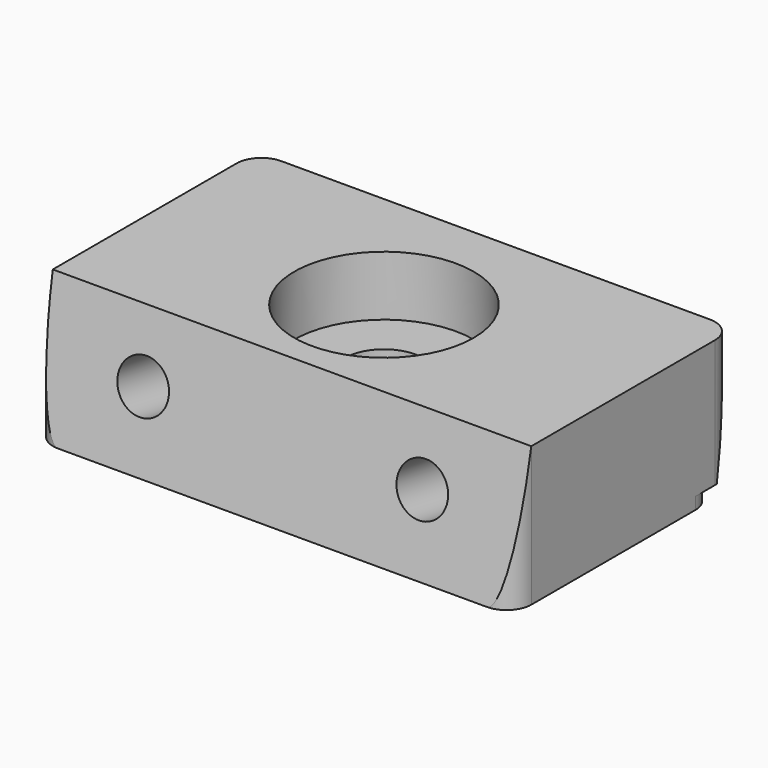
from build123d import *

# Parameters (mm, degrees)
F0_W           = 60.96
F0_H           = 35.56
F1_DEPTH       = 17.78
F2_R           = 3.175
F4_DEPTH       = 60.961
F6_D           = 10.0838
F6_DEPTH       = 23.2918
F6_CBORE_D     = 22.86
F6_CBORE_DEPTH = 7.62
F6_TIP         = 3.0294791551
F7_T1_DEPTH    = 9.4615000248
F9_D           = 6.5278
F9_DEPTH       = 23.2833333333
F9_TIP         = 1.9611489744


# Not quite as in the source:
# - a fillet or chamfer that OpenCascade refuses, or shapes differently, is made with other operations: its cross-section is extruded or revolved along the edge and cut away or added
# - a feature names something its author has since deleted; it is built from what else it names


with BuildPart() as f1:
    # F0 (on Top) → F1 (new body)
    with BuildSketch(Plane.XY):
        with Locations((30.48, 17.78)):
            Rectangle(F0_W, F0_H)
    extrude(amount=F1_DEPTH)

    # F2
    f2_edges = [f1.edges().sort_by_distance(p)[0] for p in [
        (0, 0, 8.89),
        (60.96, 0, 8.89),
        (60.96, 35.56, 8.89),
        (0, 35.56, 8.89),
    ]]
    fillet(f2_edges, radius=F2_R)

    # F3 (on face) → F4 (cut, through all)
    with BuildSketch(Plane.YZ.offset(60.96)):
        Polygon((0, 17.78), (0, 0), (3.135093717, 17.78), align=None)
        Polygon((32.424906283, 1.524), (32.424906283, 0), (35.56, 0), (35.56, 17.78), (32.6936286016, 1.524), align=None)
    extrude(amount=-F4_DEPTH, mode=Mode.SUBTRACT)

    # F6
    with Locations(Plane.XY.offset(17.78)):
        with Locations((30.4801253996, 17.78)):
            CounterBoreHole(F6_D / 2, F6_CBORE_D / 2, F6_CBORE_DEPTH, depth=F6_DEPTH)
            with Locations((0, 0, -(F6_DEPTH + F6_TIP / 2))):  # 118° drill point
                Cone(0, F6_D / 2, F6_TIP, mode=Mode.SUBTRACT)

    # F7: fillet of radius 3.175 on 2 edges, made by hand

    # F7_s2 → F7_t1 (cut)
    with BuildSketch(Plane.XY.offset(-7.9375000248)):
        with BuildLine():
            ThreePointArc((57.785, 32.424906283), (60.0300640303, 31.4949703133), (60.96, 29.249906283))
            Line((60.96, 29.249906283), (61.2775, 29.249906283))
            ThreePointArc((61.2775, 29.249906283), (61.2775, 32.385), (61.277224121, 32.4288969113))
            Line((61.277224121, 32.4288969113), (60.9597492009, 32.742406283))
            Line((60.9597492009, 32.742406283), (57.785, 32.742406283))
            Line((57.785, 32.742406283), (57.785, 32.424906283))
        make_face()
        with BuildLine():
            ThreePointArc((0, 29.249906283), (0.9299359697, 31.4949703133), (3.175, 32.424906283))
            Line((3.175, 32.424906283), (3.175, 32.742406283))
            Line((3.175, 32.742406283), (0.0002507991, 32.742406283))
            Line((0.0002507991, 32.742406283), (-0.317224121, 32.4288969113))
            ThreePointArc((-0.317224121, 32.4288969113), (-0.3175, 32.385), (-0.3175, 29.249906283))
            Line((-0.3175, 29.249906283), (0, 29.249906283))
        make_face()
    extrude(amount=F7_T1_DEPTH, mode=Mode.SUBTRACT)

    # F9
    with Locations(Plane(origin=(0, 0, 0), x_dir=(1, 0, 0), z_dir=(0, -0.984807753, 0.1736481777))):
        with Locations((12.7, 9.525), (48.26, 9.525)):
            Hole(F9_D / 2, depth=F9_DEPTH)
            with Locations((0, 0, -(F9_DEPTH + F9_TIP / 2))):  # 118° drill point
                Cone(0, F9_D / 2, F9_TIP, mode=Mode.SUBTRACT)


solid = f1.part
